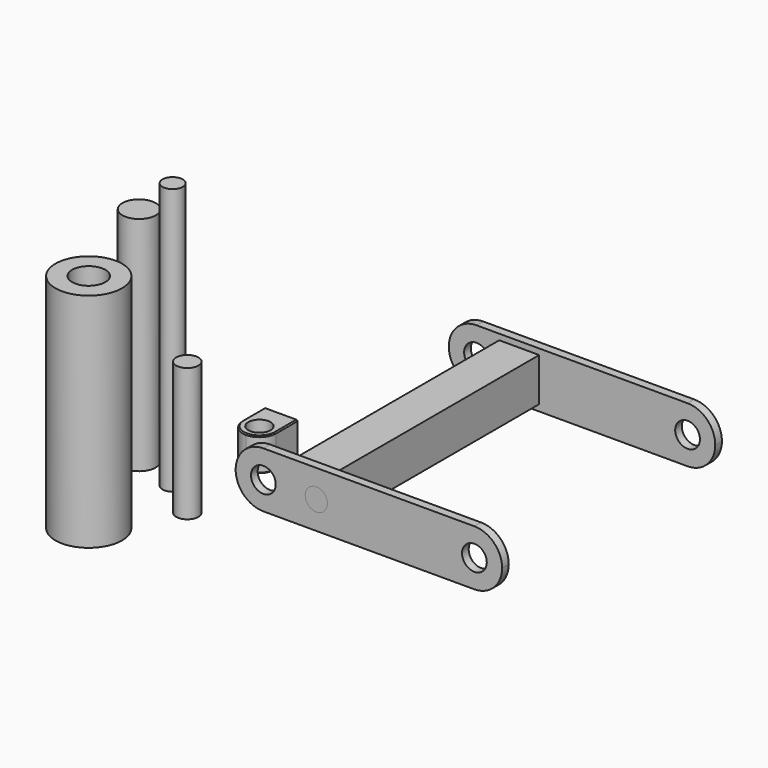
from build123d import *

# Parameters (mm, degrees)
F1_R      = 14.1536643412
F3_DEPTH  = 9.525
F2_R      = 12.7
F7_W      = 45.7254294306
F7_H      = 49.4805052876
F8_DEPTH  = 300.99
F9_R      = 11.6170502441
F10_DEPTH = 304.8
F11_R     = 38.1
F11_R_2   = 19.05
F12_DEPTH = 254
F13_DEPTH = 254
F14_R     = 12.7
F15_DEPTH = 38.1
F16_SIZE  = 1.27
F17_R     = 12.7
F18_DEPTH = 152.4


# Not quite as in the source:
# - the program builds the solid bodies; features that only make, move or delete a surface that nothing else refers to are left out


with BuildPart() as f3:
    # F1 (on face) → F3 (new body)
    with BuildSketch(Plane.XZ):
        with BuildLine():
            ThreePointArc((-15.6492135497, 111.4721251547), (-38.0998538524, 102.1727654574), (-47.3992135497, 79.7221251547))
            ThreePointArc((-47.3992135497, 79.7221251547), (-38.0998538524, 57.2714848521), (-15.6492135497, 47.9721251547))
            Line((-15.6492135497, 47.9721251547), (225.6507864503, 47.9721251547))
            ThreePointArc((225.6507864503, 47.9721251547), (248.1014267529, 57.2714848521), (257.4007864503, 79.7221251547))
            ThreePointArc((257.4007864503, 79.7221251547), (248.1014267529, 102.1727654574), (225.6507864503, 111.4721251547))
            Line((225.6507864503, 111.4721251547), (-15.6492135497, 111.4721251547))
        make_face()
        with Locations((-15.6924961424, 79.7221251547)):
            Circle(F1_R, mode=Mode.SUBTRACT)
        with Locations((225.7331678933, 79.7221251547)):
            Circle(F1_R, mode=Mode.SUBTRACT)
    extrude(amount=F3_DEPTH)


with BuildPart() as f3b:
    # F2 (on face) → F3, piece 2 (new body)
    with BuildSketch(Plane.XZ):
        with Locations((44.905539602, 79.7221251547)):
            Circle(F2_R)
    extrude(amount=F3_DEPTH)


with BuildPart() as f4_1:
    # F4: copy of F3
    add(f3.part.moved(Location((0, 304.8, 0))))


with BuildPart() as f8:
    # F7 (on face) → F8 (new body)
    with BuildSketch(Plane.XZ.offset(-295.275)):
        with Locations((33.1418430433, 80.0800956786)):
            Rectangle(F7_W, F7_H)
    extrude(amount=F8_DEPTH)


with BuildPart() as f10:
    # F9 (on Top) → F10 (new body)
    with BuildSketch(Plane.XY):
        with Locations((-167.4733012915, 50.468929112)):
            Circle(F9_R)
    extrude(amount=F10_DEPTH)


with BuildPart() as f12:
    # F11 (on Top) → F12 (new body)
    with BuildSketch(Plane.XY):
        with Locations((-174.7436672449, -60.3992268443)):
            Circle(F11_R)
        with Locations((-174.7436672449, -60.3992268443)):
            Circle(F11_R_2, mode=Mode.SUBTRACT)
    extrude(amount=F12_DEPTH)


with BuildPart() as f13:
    # F11 (on Top) → F13 (new body)
    with BuildSketch(Plane.XY):
        with Locations((-220.3151583672, 68.5483440757)):
            Circle(F11_R_2)
    extrude(amount=F13_DEPTH)


with BuildPart() as f15:
    # F14 (on Top) → F15 (new body)
    with BuildSketch(Plane.XY):
        with BuildLine():
            Line((-114.2097190022, 163.5575348735), (-152.3097190022, 163.5575348735))
            Line((-152.3097190022, 163.5575348735), (-152.3097190022, 131.8075348735))
            ThreePointArc((-152.3097190022, 131.8075348735), (-146.7301031839, 118.3371506919), (-133.2597190022, 112.7575348735))
            ThreePointArc((-133.2597190022, 112.7575348735), (-119.7893348206, 118.3371506919), (-114.2097190022, 131.8075348735))
            Line((-114.2097190022, 131.8075348735), (-114.2097190022, 163.5575348735))
        make_face()
        with Locations((-133.2597190022, 131.8075348735)):
            Circle(F14_R, mode=Mode.SUBTRACT)
    extrude(amount=F15_DEPTH)

    # F16
    f16_edges = [f15.edges().sort_by_distance(p)[0] for p in [
        (-114.209719, 147.682535, 0),
        (-133.259719, 112.757535, 0),
        (-152.309719, 147.682535, 0),
        (-133.259719, 163.557535, 0),
        (-114.209719, 163.557535, 19.05),
        (-152.309719, 163.557535, 19.05),
        (-133.259719, 163.557535, 38.1),
        (-152.309719, 147.682535, 38.1),
        (-114.209719, 147.682535, 38.1),
        (-133.259719, 112.757535, 38.1),
    ]]
    chamfer(f16_edges, length=F16_SIZE)


with BuildPart() as f18:
    # F17 (on Top) → F18 (new body)
    with BuildSketch(Plane.XY):
        with Locations((-124.5523691177, 17.8166683763)):
            Circle(F17_R)
    extrude(amount=F18_DEPTH)


solid = Compound([f3.part, f3b.part, f4_1.part, f8.part, f10.part, f12.part, f13.part, f15.part, f18.part])
